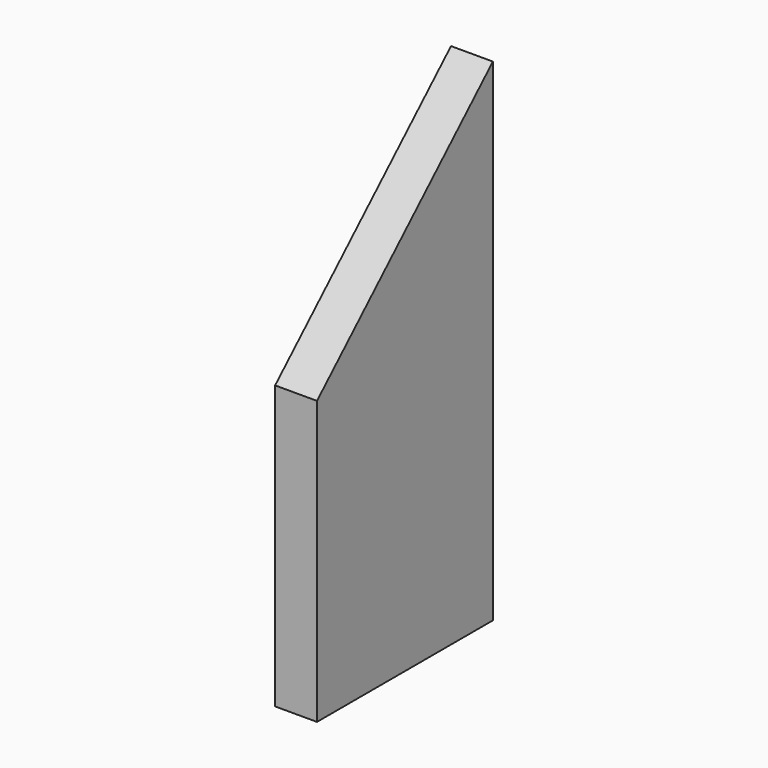
from build123d import *

# Parameters (mm, degrees)
F0_W     = 4
F0_H     = 47
F1_DEPTH = 21
F2_SIZE2 = 20.99999
F2_SIZE  = 19.99999


# Not quite as in the source:
# - a fillet or chamfer is up to 0.001 mm smaller than in the source, because OpenCascade refuses the exact size


with BuildPart() as f1:
    # F0 (on Front) → F1 (new body)
    with BuildSketch(Plane.XZ):
        Rectangle(F0_W, F0_H)
    extrude(amount=F1_DEPTH)

    # F2 (size 20 and 21 in the source; OpenCascade refuses exactly that, so slightly less here)
    f2_edges = [f1.edges().sort_by_distance(p)[0] for p in [
        (0, -21, 23.5),
    ]]
    f2_side = f1.faces().sort_by_distance((0, -21, 0))[0]
    chamfer(f2_edges, length=F2_SIZE, length2=F2_SIZE2, reference=f2_side)


solid = f1.part
